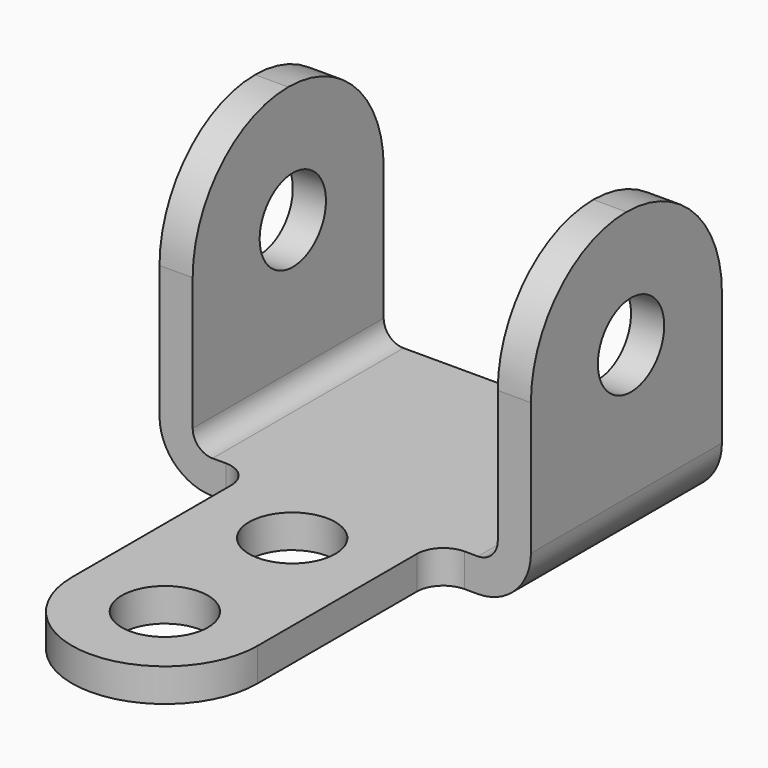
from build123d import *

# Parameters (mm, degrees)
F1_DEPTH = 57.15
F2_R     = 28.57499
F3_R     = 28.57499
F4_R     = 9.92251
F5_DEPTH = 88.901
F6_R     = 10.3251
F7_DEPTH = 7.9375


# Not quite as in the source:
# - a fillet or chamfer is up to 0.001 mm smaller than in the source, because OpenCascade refuses the exact size


with BuildPart() as f1:
    # F0 (on Front) → F1 (new body)
    with BuildSketch(Plane.XZ):
        with BuildLine():
            ThreePointArc((-44.45, 12.7), (-40.7302561211, 3.7197438789), (-31.75, 0))
            Line((-31.75, 0), (31.75, 0))
            ThreePointArc((31.75, 0), (40.7302561211, 3.7197438789), (44.45, 12.7))
            Line((44.45, 12.7), (44.45, 73.025))
            Line((44.45, 73.025), (36.5125, 73.025))
            Line((36.5125, 73.025), (36.5125, 12.7))
            ThreePointArc((36.5125, 12.7), (35.1175960454, 9.3324039546), (31.75, 7.9375))
            Line((31.75, 7.9375), (-31.75, 7.9375))
            ThreePointArc((-31.75, 7.9375), (-35.1175960454, 9.3324039546), (-36.5125, 12.7))
            Line((-36.5125, 12.7), (-36.5125, 73.025))
            Line((-36.5125, 73.025), (-44.45, 73.025))
            Line((-44.45, 73.025), (-44.45, 12.7))
        make_face()
    extrude(amount=-F1_DEPTH)

    # F2 (radius 28.575 in the source; OpenCascade refuses exactly that, so slightly less here)
    f2_edges = [f1.edges().sort_by_distance(p)[0] for p in [
        (40.48125, 0, 73.025),
        (40.48125, 57.15, 73.025),
    ]]
    fillet(f2_edges, radius=F2_R)

    # F3 (radius 28.575 in the source; OpenCascade refuses exactly that, so slightly less here)
    f3_edges = [f1.edges().sort_by_distance(p)[0] for p in [
        (-40.48125, 0, 73.025),
        (-40.48125, 57.15, 73.025),
    ]]
    fillet(f3_edges, radius=F3_R)

    # F4 (on face) → F5 (cut, through all)
    with BuildSketch(Plane(origin=(-44.45, 0, 0), x_dir=(0, -1, 0), z_dir=(-1, 0, 0))):
        with Locations((-29.956350103, 44.45)):
            Circle(F4_R)
    extrude(amount=-F5_DEPTH, mode=Mode.SUBTRACT)

    # F6 (on face) → F7 (join, through all)
    with BuildSketch(Plane.XY.offset(7.9375)):
        with BuildLine():
            Line((22.225, -53.975), (22.225, -6.35))
            ThreePointArc((22.225, -6.35), (24.0848719395, -1.8598719395), (28.575, 0))
            Line((28.575, 0), (-28.575, 0))
            ThreePointArc((-28.575, 0), (-24.0848719395, -1.8598719395), (-22.225, -6.35))
            Line((-22.225, -6.35), (-22.225, -53.975))
            ThreePointArc((-22.225, -53.975), (0, -76.2), (22.225, -53.975))
        make_face()
        with Locations((0, -53.975)):
            Circle(F6_R, mode=Mode.SUBTRACT)
        with Locations((0, -15.875)):
            Circle(F6_R, mode=Mode.SUBTRACT)
    extrude(amount=-F7_DEPTH)


solid = f1.part
